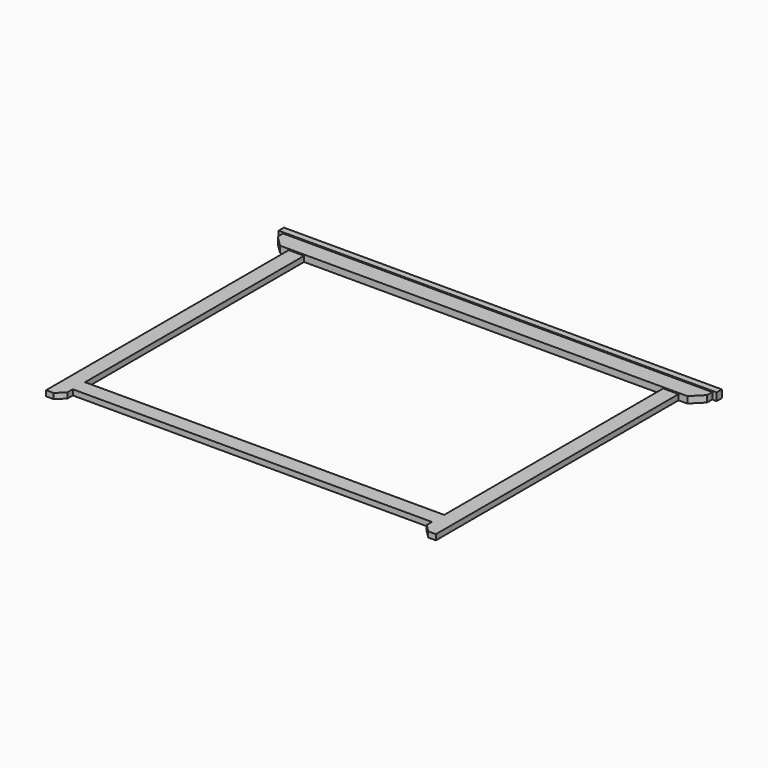
from build123d import *

# Parameters (mm, degrees)
F1_DEPTH = 30
F0_W     = 20
F0_H     = 30
F0_W_2   = 1960
F2_DEPTH = 35
F0_W_3   = 1640
F0_H_2   = 70
F3_DEPTH = 25


with BuildPart() as f1:
    # F0 (on Top) → F1 (new body)
    with BuildSketch(Plane.XY):
        Polygon((-1947.5297451019, -160.4416549206), (-1877.5297451019, -160.4416549206), (-237.5297451019, -160.4416549206), (-167.5297451019, -160.4416549206), (-127.5297451019, -160.4416549206), (-77.5297451019, -110.4416549206), (-77.5297451019, -80.4416549206), (-2037.5297451019, -80.4416549206), (-2037.5297451019, -110.4416549206), (-1987.5297451019, -160.4416549206), align=None)
    extrude(amount=F1_DEPTH)

    # F0 (on Top) → F2 (join)
    with BuildSketch(Plane.XY):
        with Locations((-2047.5297451019, -65.4416549206)):
            Rectangle(F0_W, F0_H)
        with Locations((-1057.5297451019, -65.4416549206)):
            Rectangle(F0_W_2, F0_H)
        with Locations((-67.5297451019, -65.4416549206)):
            Rectangle(F0_W, F0_H)
    extrude(amount=F2_DEPTH)

    # F0 (on Top) → F3 (join)
    with BuildSketch(Plane.XY):
        Polygon((-1877.5297451019, -1410.4416549206), (-1877.5297451019, -160.4416549206), (-1947.5297451019, -160.4416549206), (-1947.5297451019, -1545.4416549206), (-1912.5297451019, -1545.4416549206), (-1877.5297451019, -1510.4416549206), (-1877.5297451019, -1480.4416549206), align=None)
        with Locations((-1057.5297451019, -1445.4416549206)):
            Rectangle(F0_W_3, F0_H_2)
        Polygon((-167.5297451019, -160.4416549206), (-237.5297451019, -160.4416549206), (-237.5297451019, -1410.4416549206), (-237.5297451019, -1480.4416549206), (-237.5297451019, -1510.4416549206), (-202.5297451019, -1545.4416549206), (-167.5297451019, -1545.4416549206), align=None)
    extrude(amount=F3_DEPTH)


solid = f1.part
